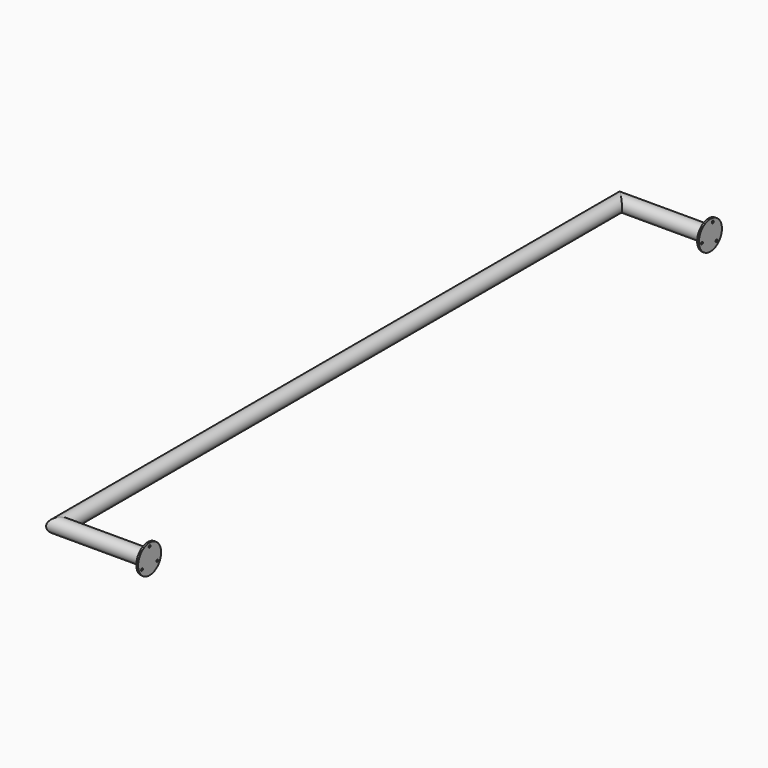
from build123d import *

# Parameters (mm, degrees)
F0_R     = 21
F0_R_2   = 20
F3_R     = 40
F3_R_2   = 3.25
F4_DEPTH = 5
F8_SIZE  = 2
F9_SIZE  = 3


with BuildPart() as f2:
    # F2: sweep along a path in F1
    with BuildLine(Plane.XY) as f2_path:
        Line((0, 0), (250, 0))
        Line((250, 0), (250, -1948.319))
        Line((250, -1948.319), (0, -1948.319))
    # F0 (on Right) → F2 (sweep)
    with BuildSketch(Plane.YZ):
        Circle(F0_R)
        Circle(F0_R_2, mode=Mode.SUBTRACT)
    sweep(path=f2_path.line, transition=Transition.RIGHT)

    # F3 (on face) → F4 (join)
    with BuildSketch(Plane(origin=(0, 0, 0), x_dir=(0, -1, 0), z_dir=(-1, 0, 0))):
        with Locations((1948.319, 0)):
            Circle(F3_R)
        with Locations((1921.9052251846, -15.25)):
            Circle(F3_R_2, mode=Mode.SUBTRACT)
        with Locations((1974.7327748154, -15.25)):
            Circle(F3_R_2, mode=Mode.SUBTRACT)
        with Locations((1948.319, 30.5)):
            Circle(F3_R_2, mode=Mode.SUBTRACT)
        Circle(F3_R)
        with Locations((-21.187080299, -21.9398639103)):
            Circle(F3_R_2, mode=Mode.SUBTRACT)
        with Locations((29.5940196514, -7.3786178158)):
            Circle(F3_R_2, mode=Mode.SUBTRACT)
        with Locations((-8.4069393524, 29.3184817261)):
            Circle(F3_R_2, mode=Mode.SUBTRACT)
    extrude(amount=-F4_DEPTH)


with BuildPart() as f6_1:
    # F6: instance of F2
    add(f2.part.mirror(Plane(origin=(-25, 0, 0), x_dir=(0, -1, 0), z_dir=(-1, 0, 0))))

    # F8
    f8_edges = [f6_1.edges().sort_by_distance(p)[0] for p in [
        (-55, -1945.069, 30.5),
        (-55, -1918.655225, -15.25),
        (-55, -1971.482775, -15.25),
        (-55, 11.656939, 29.318482),
        (-55, -26.34402, -7.378618),
        (-55, 24.43708, -21.939864),
    ]]
    chamfer(f8_edges, length=F8_SIZE)

    # F9
    f9_edges = [f6_1.edges().sort_by_distance(p)[0] for p in [
        (-55, -21, 0),
        (-55, -1927.319, 0),
    ]]
    chamfer(f9_edges, length=F9_SIZE)


solid = f6_1.part
